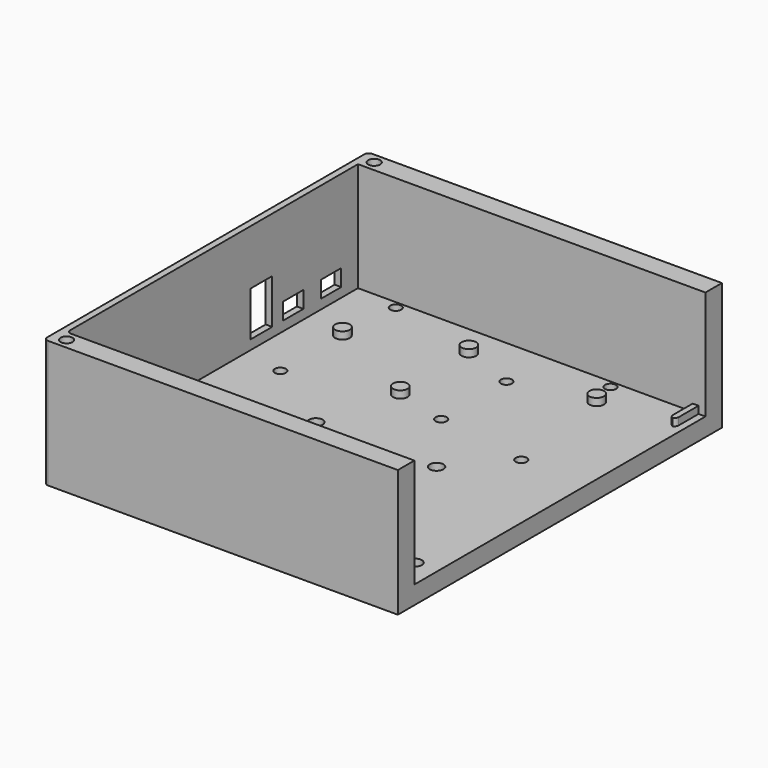
from build123d import *

# Parameters (mm, degrees)
F5_W         = 192.786
F5_H         = 141.3764
F7_DEPTH     = 44.45
F12_W        = 187.452
F12_H        = 127
F14_DEPTH    = 38.1
F4_R         = 15.621
F4_R_2       = 13.081
F13_W        = 2.032
F13_H        = 10.16
F13_W_2      = 10.16
F13_H_2      = 2.032
F15_DEPTH    = 8.89
F16_DEPTH    = 2.9972
F17_DEPTH    = 3.81
F10_R        = 2.3749
F18_DEPTH    = 25.4
F3_R         = 1.9304
F19_DEPTH    = 25.4
F11_R        = 2.54
F20_DEPTH    = 8.89
F21_W        = 8.89
F21_H        = 5.842
F21_W_2      = 9.525
F21_H_2      = 15.621
F22_DEPTH    = 25.4
F23_R        = 2.0828
F24_DEPTH    = 4.318
F25_T1_DEPTH = 41.91
F25_T3_DEPTH = 52.07
F25_T5_DEPTH = 6.35
F26_W        = 69.2167831277
F26_H        = 141.3764
F27_DEPTH    = 50.8


# Not quite as in the source:
# - a fillet or chamfer that OpenCascade refuses, or shapes differently, is made with other operations: its cross-section is extruded or revolved along the edge and cut away or added


with BuildPart() as f7:
    # F5 (on Top) → F7 (new body)
    with BuildSketch(Plane.XY):
        with Locations((-4.773771323, -23.1295908162)):
            Rectangle(F5_W, F5_H)
    extrude(amount=F7_DEPTH)

    # F12 (on face) → F14 (cut)
    with BuildSketch(Plane.XY.offset(44.45)):
        with Locations((-5.154771323, -23.1295908162)):
            Rectangle(F12_W, F12_H)
    extrude(amount=-F14_DEPTH, mode=Mode.SUBTRACT)

    # F4 (on Top) + F13 (on Top) → F15 (join)
    with BuildSketch(Plane.XY):
        with Locations((-81.989771323, -51.9585908162)):
            Circle(F4_R)
        with Locations((-81.989771323, -51.9585908162)):
            Circle(F4_R_2, mode=Mode.SUBTRACT)
    with BuildSketch(Plane.XY):
        with Locations((18.975228677, 35.2904091838)):
            Rectangle(F13_W, F13_H)
        with Locations((47.6495291469, -25.7965908162)):
            Rectangle(F13_W_2, F13_H_2)
    extrude(amount=F15_DEPTH)

    # F6 (on face) → F16 (cut)
    with BuildSketch(Plane.XY):
        Polygon((-81.6243755079, 34.3379091838), (-79.6079796927, 37.8304091838), (-81.6243755079, 41.3229091838), (-85.6571671382, 41.3229091838), (-87.6735629533, 37.8304091838), (-85.6571671382, 34.3379091838), align=None)
        Polygon((-6.6943755079, 34.3379091838), (-4.6779796927, 37.8304091838), (-6.6943755079, 41.3229091838), (-10.7271671382, 41.3229091838), (-12.7435629533, 37.8304091838), (-10.7271671382, 34.3379091838), align=None)
        Polygon((-30.8243755079, 19.0979091838), (-28.8079796927, 22.5904091838), (-30.8243755079, 26.0829091838), (-34.8571671382, 26.0829091838), (-36.8735629533, 22.5904091838), (-34.8571671382, 19.0979091838), align=None)
        Polygon((-82.8943755079, -14.4300908162), (-80.8779796927, -10.9375908162), (-82.8943755079, -7.4450908162), (-86.9271671382, -7.4450908162), (-88.9435629533, -10.9375908162), (-86.9271671382, -14.4300908162), align=None)
        Polygon((-30.8243755079, -9.3500908162), (-28.8079796927, -5.8575908162), (-30.8243755079, -2.3650908162), (-34.8571671382, -2.3650908162), (-36.8735629533, -5.8575908162), (-34.8571671382, -9.3500908162), align=None)
        Polygon((1.1796244921, -14.4300908162), (3.1960203073, -10.9375908162), (1.1796244921, -7.4450908162), (-2.8531671382, -7.4450908162), (-4.8695629533, -10.9375908162), (-2.8531671382, -14.4300908162), align=None)
    extrude(amount=F16_DEPTH, mode=Mode.SUBTRACT)

    # F9 (on Top) → F17 (cut)
    with BuildSketch(Plane.XY):
        Polygon((-55.7338586688, -33.239207965), (-53.0355544507, -28.565607965), (-55.7338586688, -23.892007965), (-61.130467105, -23.892007965), (-63.828771323, -28.565607965), (-61.130467105, -33.239207965), align=None)
        Polygon((-24.9998586688, -81.067407965), (-22.3015544507, -76.393807965), (-24.9998586688, -71.720207965), (-30.396467105, -71.720207965), (-33.094771323, -76.393807965), (-30.396467105, -81.067407965), align=None)
        Polygon((17.1641413312, -71.720207965), (14.4658371131, -71.720207965), (11.767532895, -71.720207965), (9.069228677, -76.393807965), (11.767532895, -81.067407965), (17.1641413312, -81.067407965), (19.8624455493, -76.393807965), align=None)
        Polygon((-10.8715544507, -28.565607965), (-13.5698586688, -23.892007965), (-18.966467105, -23.892007965), (-21.664771323, -28.565607965), (-18.966467105, -33.239207965), (-13.5698586688, -33.239207965), align=None)
    extrude(amount=F17_DEPTH, mode=Mode.SUBTRACT)

    # F10 (on Top) → F18 (cut)
    with BuildSketch(Plane.XY):
        with Locations((-58.4321628869, -28.565607965)):
            Circle(F10_R)
        with Locations((-27.6981628869, -76.393807965)):
            Circle(F10_R)
        with Locations((-16.2681628869, -28.565607965)):
            Circle(F10_R)
        with Locations((14.4658371131, -76.393807965)):
            Circle(F10_R)
    extrude(amount=F18_DEPTH, mode=Mode.SUBTRACT)

    # F3 (on Top) → F19 (cut)
    with BuildSketch(Plane.XY):
        with Locations((-84.910771323, -10.9375908162)):
            Circle(F3_R)
        with Locations((-32.840771323, -5.8575908162)):
            Circle(F3_R)
        with Locations((-32.840771323, 22.5904091838)):
            Circle(F3_R)
        with Locations((-8.710771323, 37.8304091838)):
            Circle(F3_R)
        with Locations((-83.640771323, 37.8304091838)):
            Circle(F3_R)
        with Locations((-0.836771323, -10.9375908162)):
            Circle(F3_R)
    extrude(amount=F19_DEPTH, mode=Mode.SUBTRACT)

    # F11 (on Top) → F20 (join)
    with BuildSketch(Plane.XY):
        with Locations((-6.1370921321, 28.5807047039)):
            Circle(F11_R)
        with Locations((-51.3140404916, 29.3099723562)):
            Circle(F11_R)
        with Locations((-50.6939233637, -1.3771463051)):
            Circle(F11_R)
        with Locations((-84.7697969953, 15.9851294398)):
            Circle(F11_R)
    extrude(amount=F20_DEPTH)

    # F21 (on face) → F22 (cut)
    with BuildSketch(Plane(origin=(-101.166771323, 0, 0), x_dir=(0, -1, 0), z_dir=(-1, 0, 0))):
        with Locations((-12.1256091838, 12.573)):
            Rectangle(F21_W, F21_H)
        with Locations((-28.6356091838, 12.573)):
            Rectangle(F21_W, F21_H)
        with Locations((1.7808908162, 17.4625)):
            Rectangle(F21_W_2, F21_H_2)
    extrude(amount=-F22_DEPTH, mode=Mode.SUBTRACT)

    # F23 (on face) → F24 (cut)
    with BuildSketch(Plane.XY.offset(44.45)):
        with Locations((-96.086771323, -90.2236908162)):
            Circle(F23_R)
        with Locations((86.539228677, -90.2236908162)):
            Circle(F23_R)
        with Locations((86.539228677, 43.9645091838)):
            Circle(F23_R)
        with Locations((-96.086771323, 43.9645091838)):
            Circle(F23_R)
    extrude(amount=-F24_DEPTH, mode=Mode.SUBTRACT)

    # F25: fillet of radius 1.524 on 12 edges, made by hand

    # F25_s2 → F25_t1 (join)
    with BuildSketch(Plane.XY.offset(2.54)):
        with BuildLine():
            ThreePointArc((-97.356771323, -86.6295908162), (-98.4344020576, -86.1832215507), (-98.880771323, -85.1055908162))
            Line((-98.880771323, -85.1055908162), (-98.880771323, -86.6295908162))
            Line((-98.880771323, -86.6295908162), (-97.356771323, -86.6295908162))
        make_face()
        with BuildLine():
            ThreePointArc((88.571228677, -85.1055908162), (88.1248594115, -86.1832215507), (87.047228677, -86.6295908162))
            Line((87.047228677, -86.6295908162), (88.571228677, -86.6295908162))
            Line((88.571228677, -86.6295908162), (88.571228677, -85.1055908162))
        make_face()
    extrude(amount=F25_T1_DEPTH)

    # F25_s4 → F25_t3 (cut)
    with BuildSketch(Plane.XY.offset(-3.81)):
        with BuildLine():
            ThreePointArc((-99.642771323, 47.5586091838), (-100.7204020576, 47.1122399184), (-101.166771323, 46.0346091838))
            Line((-101.166771323, 46.0346091838), (-101.166771323, 47.5586091838))
            Line((-101.166771323, 47.5586091838), (-99.642771323, 47.5586091838))
        make_face()
        with BuildLine():
            ThreePointArc((-101.166771323, -92.2937908162), (-100.7204020576, -93.3714215507), (-99.642771323, -93.8177908162))
            Line((-99.642771323, -93.8177908162), (-101.166771323, -93.8177908162))
            Line((-101.166771323, -93.8177908162), (-101.166771323, -92.2937908162))
        make_face()
        with BuildLine():
            ThreePointArc((91.619228677, -92.2937908162), (91.1728594115, -93.3714215507), (90.095228677, -93.8177908162))
            Line((90.095228677, -93.8177908162), (91.619228677, -93.8177908162))
            Line((91.619228677, -93.8177908162), (91.619228677, -92.2937908162))
        make_face()
        with BuildLine():
            ThreePointArc((90.095228677, 47.5586091838), (91.1728594115, 47.1122399184), (91.619228677, 46.0346091838))
            Line((91.619228677, 46.0346091838), (91.619228677, 47.5586091838))
            Line((91.619228677, 47.5586091838), (90.095228677, 47.5586091838))
        make_face()
    extrude(amount=F25_T3_DEPTH, mode=Mode.SUBTRACT)

    # F25_s6 → F25_t5 (cut)
    with BuildSketch(Plane.XY.offset(6.35)):
        with BuildLine():
            ThreePointArc((17.959228677, 31.7344091838), (18.4055979424, 30.6567784493), (19.483228677, 30.2104091838))
            Line((19.483228677, 30.2104091838), (17.959228677, 30.2104091838))
            Line((17.959228677, 30.2104091838), (17.959228677, 31.7344091838))
        make_face()
        with BuildLine():
            ThreePointArc((42.5695291469, -25.2885908162), (43.0158984124, -26.3662215507), (44.0935291469, -26.8125908162))
            Line((44.0935291469, -26.8125908162), (42.5695291469, -26.8125908162))
            Line((42.5695291469, -26.8125908162), (42.5695291469, -25.2885908162))
        make_face()
        with BuildLine():
            ThreePointArc((42.5695291469, -26.3045908162), (43.0158984124, -25.2269600816), (44.0935291469, -24.7805908162))
            Line((44.0935291469, -24.7805908162), (42.5695291469, -24.7805908162))
            Line((42.5695291469, -24.7805908162), (42.5695291469, -26.3045908162))
        make_face()
        with BuildLine():
            ThreePointArc((19.991228677, 31.7344091838), (19.5448594115, 30.6567784493), (18.467228677, 30.2104091838))
            Line((18.467228677, 30.2104091838), (19.991228677, 30.2104091838))
            Line((19.991228677, 30.2104091838), (19.991228677, 31.7344091838))
        make_face()
        with BuildLine():
            ThreePointArc((51.2055291469, -26.8125908162), (52.2831598814, -26.3662215507), (52.7295291469, -25.2885908162))
            Line((52.7295291469, -25.2885908162), (52.7295291469, -26.8125908162))
            Line((52.7295291469, -26.8125908162), (51.2055291469, -26.8125908162))
        make_face()
        with BuildLine():
            ThreePointArc((51.2055291469, -24.7805908162), (52.2831598814, -25.2269600816), (52.7295291469, -26.3045908162))
            Line((52.7295291469, -26.3045908162), (52.7295291469, -24.7805908162))
            Line((52.7295291469, -24.7805908162), (51.2055291469, -24.7805908162))
        make_face()
    extrude(amount=F25_T5_DEPTH, mode=Mode.SUBTRACT)

    # F26 (on Top) → F27 (cut)
    with BuildSketch(Plane.XY):
        with Locations((57.0108371131, -23.1295908162)):
            Rectangle(F26_W, F26_H)
    extrude(amount=F27_DEPTH, mode=Mode.SUBTRACT)


solid = f7.part
